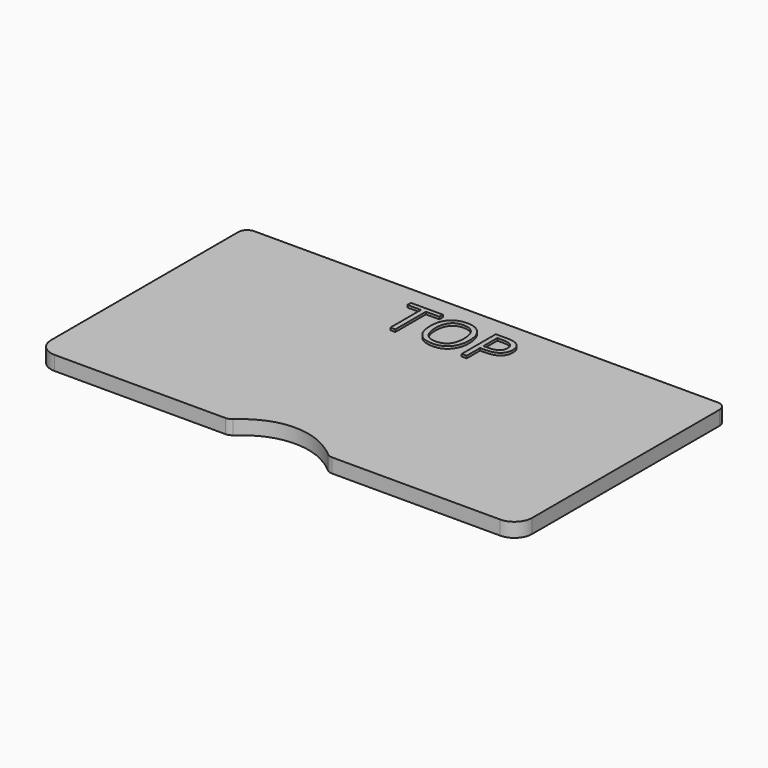
from build123d import *

# Parameters (mm, degrees)
F1_DEPTH     = 1.524
F2_R         = 0.9525
F3_R         = 1.905
F4_TEXT_SIZE = 6.3966959715
F5_DEPTH     = 0.254


# Not quite as in the source:
# - Text() gives the source's letters only with a copy of the font that has no kerning and outlines rounded to 1/6400 em; it was checked with that copy


with BuildPart() as f1:
    # F0 (on Top) → F1 (new body)
    with BuildSketch(Plane.XY):
        with BuildLine():
            Line((-25.781, 13.97), (-25.781, -13.97))
            Line((-25.781, -13.97), (-5.1949317567, -13.97))
            add(Edge.make_bspline(
                [(-5.1949317567, -13.97), (-3.4827579036, -12.3440297914), (0.0036350037, -11.0380310877), (3.6538117697, -12.3147736347), (5.511269439, -13.97)],
                knots=[0, 0, 0, 0, 0.4937522698, 1, 1, 1, 1], degree=3))
            Line((5.511269439, -13.97), (25.781, -13.97))
            Line((25.781, -13.97), (25.781, 13.97))
            Line((25.781, 13.97), (-25.781, 13.97))
        make_face()
    extrude(amount=F1_DEPTH)

    # F2
    f2_edges = [f1.edges().sort_by_distance(p)[0] for p in [
        (-25.781, 13.97, 0.762),
        (25.781, 13.97, 0.762),
        (-5.194932, -13.97, 0.762),
        (5.511269, -13.97, 0.762),
    ]]
    fillet(f2_edges, radius=F2_R)

    # F3
    f3_edges = [f1.edges().sort_by_distance(p)[0] for p in [
        (25.781, -13.97, 0.762),
        (-25.781, -13.97, 0.762),
    ]]
    fillet(f3_edges, radius=F3_R)

    # F4 (on face) → F5 (join)
    with BuildSketch(Plane.XY.offset(1.524)):
        with Locations((-6.2292824441, 7.0737572387)):
            Text('TOP', F4_TEXT_SIZE, font='Open Sans', text_align=(TextAlign.LEFT, TextAlign.BOTTOM))
    extrude(amount=F5_DEPTH)


solid = f1.part
